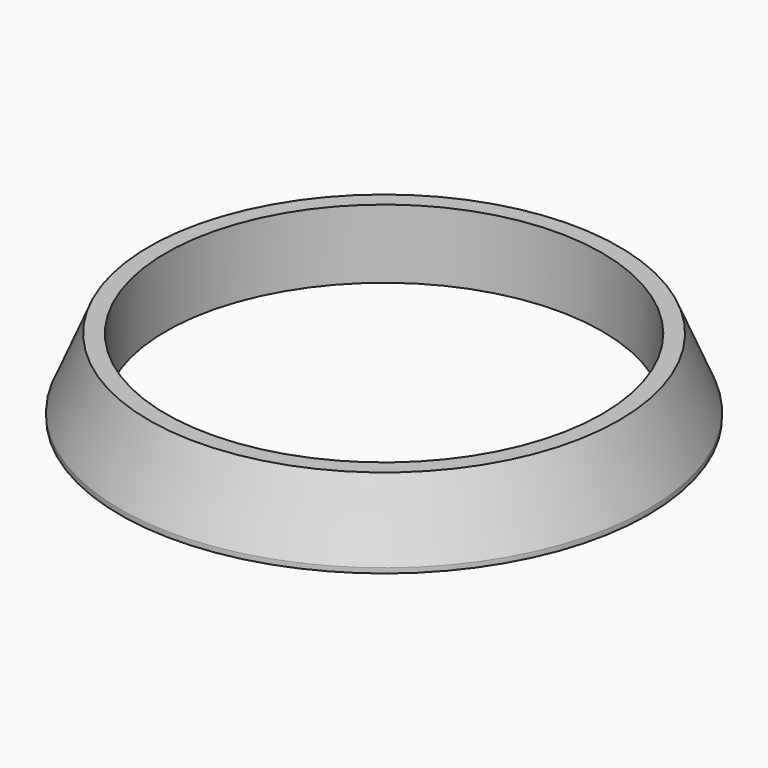
from build123d import *

# Parameters (mm, degrees)
F2_SIZE2 = 1.99898
F2_SIZE  = 4.7625


# Not quite as in the source:
# - a feature of the source that left no trace in its solid (it failed there, or was rolled back) is left out


with BuildPart() as f1:
    # F0 (on Front) → F1 (revolve)
    with BuildSketch(Plane.XZ):
        with BuildLine():
            ThreePointArc((15.08252, 24.6518301586), (16.6709354351, 24.485444554), (18.25752, 24.3024221995))
            Line((18.25752, 24.3024221995), (18.25752, 29.4143301586))
            Line((18.25752, 29.4143301586), (15.08252, 29.4143301586))
            Line((15.08252, 29.4143301586), (15.08252, 24.6518301586))
        make_face()
    revolve(axis=Axis((0, 0, 31.4977962196), (0, 0, 1)))

    # F2
    f2_edges = [f1.edges().sort_by_distance(p)[0] for p in [
        (-18.25752, 0, 29.41433),
    ]]
    chamfer(f2_edges, length=F2_SIZE, length2=F2_SIZE2)


solid = f1.part
